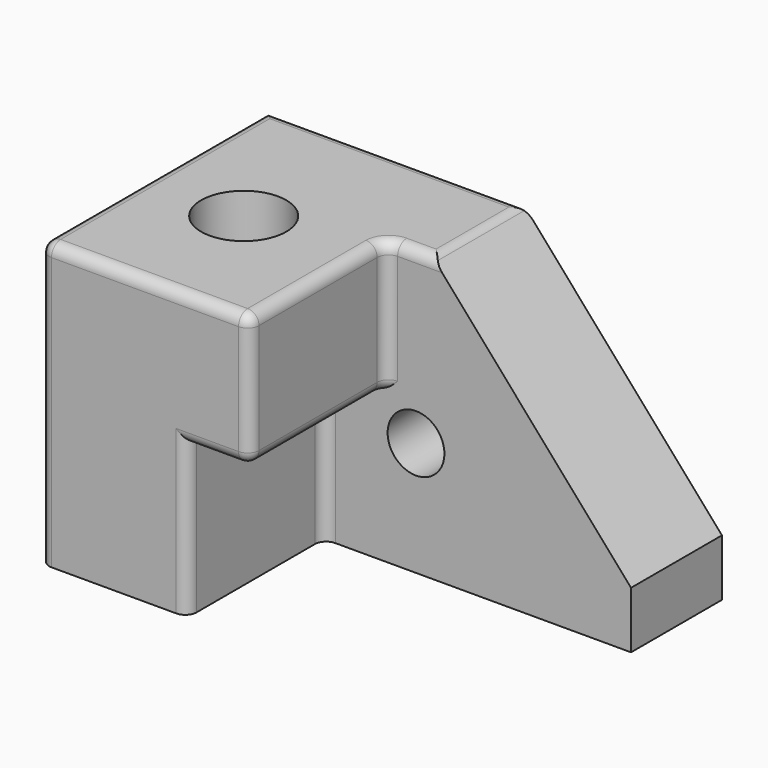
from build123d import *

# Parameters (mm, degrees)
F0_W         = 203.2
F0_H         = 127
F1_DEPTH     = 127
F3_DEPTH     = 76.2
F4_SIZE2     = 101.6
F4_SIZE      = 88.9
F5_F1_R      = 5.08
F5_F2_R      = 5.08
F6_T1_DEPTH  = 66.04
F6_S5_W      = 5.1816
F6_S5_H      = 5.1816
F6_T6_DEPTH  = 5.1816
F6_T12_ANGLE = 233.2969892374
F7_R         = 12.7
F8_DEPTH     = 50.801
F9_R         = 19.05
F10_DEPTH    = 127.0010001


# Not quite as in the source:
# - a fillet or chamfer that OpenCascade refuses, or shapes differently, is made with other operations: its cross-section is extruded or revolved along the edge and cut away or added


with BuildPart() as f1:
    # F0 (on Front) → F1 (new body)
    with BuildSketch(Plane.XZ):
        with Locations((13.6157348752, 8.31202526)):
            Rectangle(F0_W, F0_H)
    extrude(amount=F1_DEPTH)

    # F2 (on face) → F3 (cut)
    with BuildSketch(Plane.XZ.offset(127)):
        Polygon((115.2157348752, 71.81202526), (5.7971677743, 71.81202526), (5.7971677743, 12.5097064301), (-22.089054808, 12.5097064301), (-22.089054808, -55.18797474), (115.2157348752, -55.18797474), align=None)
    extrude(amount=-F3_DEPTH, mode=Mode.SUBTRACT)

    # F4
    f4_edges = [f1.edges().sort_by_distance(p)[0] for p in [
        (115.215735, -25.4, 71.812025),
    ]]
    f4_side = f1.faces().sort_by_distance((-8.764887, -51.376752, 71.812025))[0]
    chamfer(f4_edges, length=F4_SIZE, length2=F4_SIZE2, reference=f4_side)

    # F5: fillet of radius 5.08 on 11 edges, made by hand

    # F5_f1
    f5_f1_edges = [f1.edges().sort_by_distance(p)[0] for p in [
        (5.7971677743, -50.8, 42.1608658451),
        (-22.089054808, -50.8, -21.3391341549),
    ]]
    fillet(f5_f1_edges, radius=F5_F1_R)

    # F5_f2
    f5_f2_edges = [f1.edges().sort_by_distance(p)[0] for p in [
        (5.7971677743, -91.44, 71.81202526),
        (5.7971677743, -127, 42.1608658451),
        (26.3157348752, -25.4, 71.81202526),
        (-30.8342651248, 0, 71.81202526),
        (-87.9842651248, -63.5, 71.81202526),
        (-8.1459435169, -127, 12.5097064301),
        (-22.089054808, -127, -21.3391341549),
        (-87.9842651248, -127, 8.31202526),
        (-41.0935486753, -127, 71.81202526),
        (7.2850653259, -52.2878975516, 71.81202526),
    ]]
    fillet(f5_f2_edges, radius=F5_F2_R)

    # F6: fillet of radius 5.08 on 2 edges, made by hand

    # F6_s2 → F6_t1 (cut)
    with BuildSketch(Plane.XZ.offset(55.88)):
        with BuildLine():
            ThreePointArc((5.7971677743, 17.5897064301), (4.3092702227, 13.9976039817), (0.7171677743, 12.5097064301))
            Line((0.7171677743, 12.5097064301), (5.7971677743, 12.5097064301))
            Line((5.7971677743, 12.5097064301), (5.7971677743, 17.5897064301))
        make_face()
    extrude(amount=F6_T1_DEPTH, mode=Mode.SUBTRACT)


with BuildPart() as f6_tool4:
    # F6_s5 → F6_t6 (new body)
    with BuildSketch(Plane.YZ.offset(0.7171677743)):
        with Locations((-124.5108, 14.9989064301)):
            Rectangle(F6_S5_W, F6_S5_H)
    extrude(amount=F6_T6_DEPTH)

    # F6_s7 → F6_t8 (revolve, cut)
    with BuildSketch(Plane(origin=(0.7171677743, -121.92, 17.5897064301), x_dir=(0, 0.7071067812, 0.7071067812), z_dir=(0, 0.7071067812, -0.7071067812))):
        with BuildLine():
            ThreePointArc((0, -5.08), (5.08, 0), (0, 5.08))
            Line((0, 5.08), (0, -5.08))
        make_face()
    revolve(axis=Axis((0.7171677743, -121.92, 17.5897064301), (1, 0, 0)), mode=Mode.SUBTRACT)


with BuildPart() as f1_1:
    add(f1.part)

    # F6_t3: cut F6_tool4
    add(f6_tool4.part, mode=Mode.SUBTRACT)


with BuildPart() as f6_tool10:
    # F6_s11 → F6_t12 (revolve)
    with BuildSketch(Plane(origin=(-19.784595187, -14.7486000708, 0), x_dir=(0, 0, 1), z_dir=(-0.8017442393, -0.5976672776, 0))):
        with BuildLine():
            ThreePointArc((17.5897064301, -56.382395344), (13.9976039817, -57.8702928955), (12.5097064301, -61.462395344))
            Line((12.5097064301, -61.462395344), (12.5097064301, -56.382395344))
            Line((12.5097064301, -56.382395344), (17.5897064301, -56.382395344))
        make_face()
    revolve(axis=Axis((10.8771677743, -55.88, 12.5097064301), (0, 0, 1)), revolution_arc=F6_T12_ANGLE)

    split(bisect_by=Plane.XZ.offset(50.8), keep=Keep.TOP)


with BuildPart() as f1_2:
    add(f1_1.part)

    # F6_t9: cut F6_tool10
    add(f6_tool10.part, mode=Mode.SUBTRACT)

    # F7 (on face) → F8 (cut, through all)
    with BuildSketch(Plane.XZ.offset(50.8)):
        with Locations((19.088730216, -4.1699022986)):
            Circle(F7_R)
    extrude(amount=-F8_DEPTH, mode=Mode.SUBTRACT)

    # F9 (on face) → F10 (cut, through all)
    with BuildSketch(Plane.XY.offset(71.81202526)):
        with Locations((-44.067915529, -68.1414976716)):
            Circle(F9_R)
    extrude(amount=-F10_DEPTH, mode=Mode.SUBTRACT)


solid = f1_2.part
